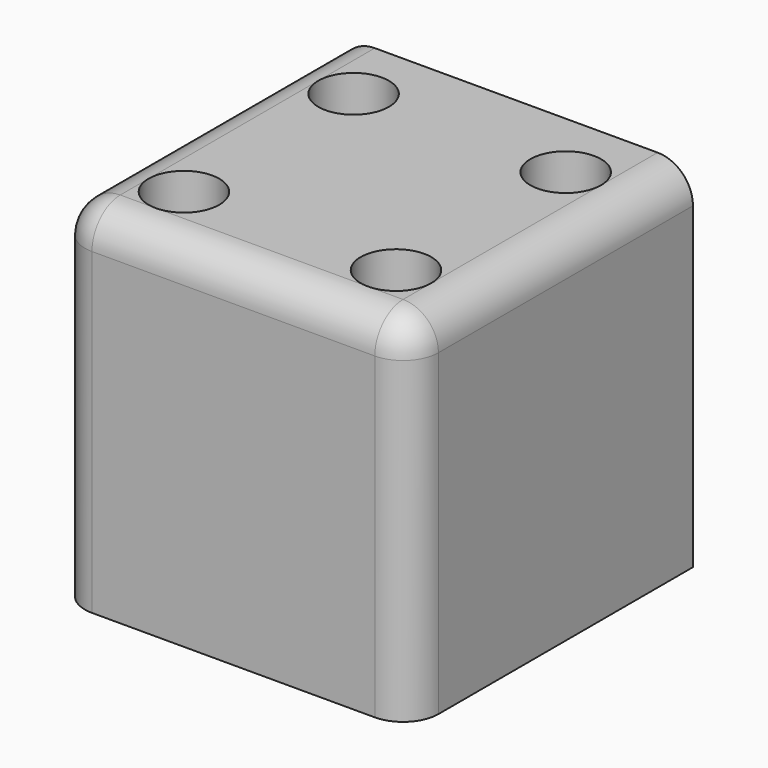
from build123d import *

# Parameters (mm, degrees)
F0_W     = 50
F0_H     = 50
F0_R     = 5
F0_R_2   = 2.5
F1_DEPTH = 50
F2_START = 10
F2_DEPTH = 40
F3_R     = 4.99999
F4_R     = 10
F5_DEPTH = 10


# Not quite as in the source:
# - a fillet or chamfer is up to 0.001 mm smaller than in the source, because OpenCascade refuses the exact size


with BuildPart() as f1:
    # F0 (on Top) → F1 (new body)
    with BuildSketch(Plane.XY):
        Rectangle(F0_W, F0_H)
        with Locations((-15, -15)):
            Circle(F0_R, mode=Mode.SUBTRACT)
        with Locations((15, -15)):
            Circle(F0_R, mode=Mode.SUBTRACT)
        with Locations((-15, 15)):
            Circle(F0_R, mode=Mode.SUBTRACT)
        with Locations((15, 15)):
            Circle(F0_R, mode=Mode.SUBTRACT)
        with Locations((-15, -15)):
            Circle(F0_R)
        with Locations((-15, -15)):
            Circle(F0_R_2, mode=Mode.SUBTRACT)
        with Locations((-15, 15)):
            Circle(F0_R)
        with Locations((-15, 15)):
            Circle(F0_R_2, mode=Mode.SUBTRACT)
        with Locations((15, 15)):
            Circle(F0_R)
        with Locations((15, 15)):
            Circle(F0_R_2, mode=Mode.SUBTRACT)
        with Locations((15, -15)):
            Circle(F0_R)
        with Locations((15, -15)):
            Circle(F0_R_2, mode=Mode.SUBTRACT)
    extrude(amount=F1_DEPTH)

    # F0 (on Top) → F2 (cut)
    with BuildSketch(Plane.XY.offset(F2_START)):
        with Locations((-15, -15)):
            Circle(F0_R)
        with Locations((-15, -15)):
            Circle(F0_R_2, mode=Mode.SUBTRACT)
        with Locations((-15, 15)):
            Circle(F0_R)
        with Locations((-15, 15)):
            Circle(F0_R_2, mode=Mode.SUBTRACT)
        with Locations((15, -15)):
            Circle(F0_R)
        with Locations((15, -15)):
            Circle(F0_R_2, mode=Mode.SUBTRACT)
        with Locations((15, 15)):
            Circle(F0_R)
        with Locations((15, 15)):
            Circle(F0_R_2, mode=Mode.SUBTRACT)
    extrude(amount=F2_DEPTH, mode=Mode.SUBTRACT)

    # F3 (radius 5 in the source; OpenCascade refuses exactly that, so slightly less here)
    f3_edges = [f1.edges().sort_by_distance(p)[0] for p in [
        (-25, -25, 25),
        (25, -25, 25),
        (0, -25, 50),
        (-25, 0, 50),
        (25, 0, 50),
    ]]
    fillet(f3_edges, radius=F3_R)

    # F4 (on face) → F5 (join)
    with BuildSketch(Plane(origin=(0, 25, 0), x_dir=(-1, 0, 0), z_dir=(0, 1, 0))):
        with Locations((0, 22.5)):
            Circle(F4_R)
    extrude(amount=F5_DEPTH)


solid = f1.part
